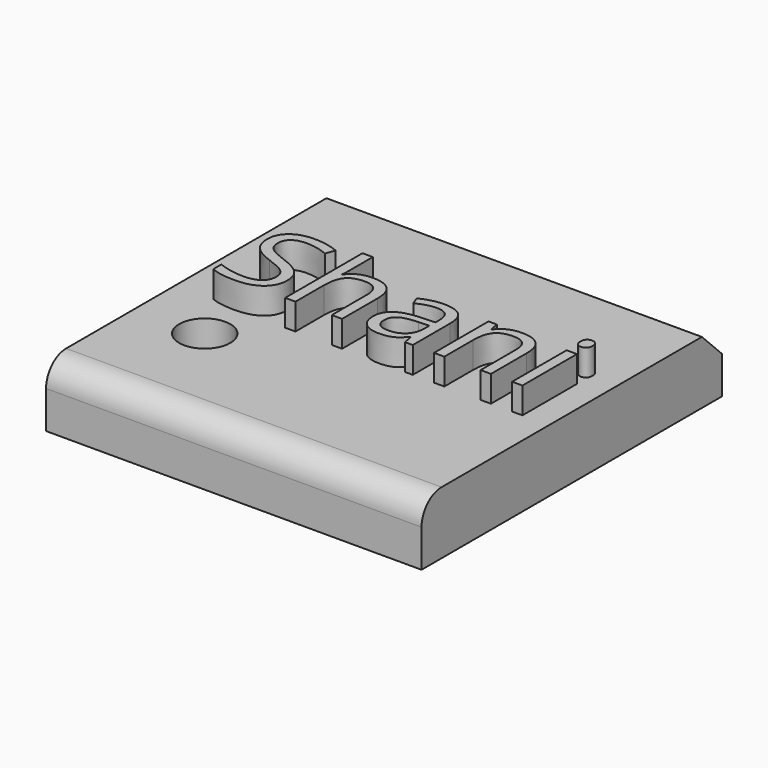
from build123d import *

# Parameters (mm, degrees)
F0_W         = 76.2
F0_H         = 76.2
F1_DEPTH     = 12.7
F2_TEXT_SIZE = 25.8248231451
F3_DEPTH     = 5.334
F4_R         = 5.08
F5_R         = 5.1865093995
F6_DEPTH     = 25.4
F7_SIZE      = 5.08


# Not quite as in the source:
# - Text() gives the source's letters only with a copy of the font that has no kerning and outlines rounded to 1/6400 em; it was checked with that copy


with BuildPart() as f1:
    # F0 (on Top) → F1 (new body)
    with BuildSketch(Plane.XY):
        with Locations((-12.0710246265, 9.1704332528)):
            Rectangle(F0_W, F0_H)
    extrude(amount=F1_DEPTH)

    # F2 (on face) → F3 (join)
    with BuildSketch(Plane.XY.offset(12.7)):
        with Locations((-43.9059901983, 3.3950631041)):
            Text('Shani', F2_TEXT_SIZE, font='Open Sans', text_align=(TextAlign.LEFT, TextAlign.BOTTOM))
    extrude(amount=F3_DEPTH)

    # F4
    f4_edges = [f1.edges().sort_by_distance(p)[0] for p in [
        (-12.071025, -28.929567, 12.7),
    ]]
    fillet(f4_edges, radius=F4_R)

    # F5 (on face) → F6 (cut)
    with BuildSketch(Plane.XY.offset(12.7)):
        with Locations((-36.2182371318, -6.124726031)):
            Circle(F5_R)
    extrude(amount=-F6_DEPTH, mode=Mode.SUBTRACT)

    # F7
    f7_edges = [f1.edges().sort_by_distance(p)[0] for p in [
        (-12.071025, 47.270433, 12.7),
    ]]
    chamfer(f7_edges, length=F7_SIZE)


solid = f1.part
